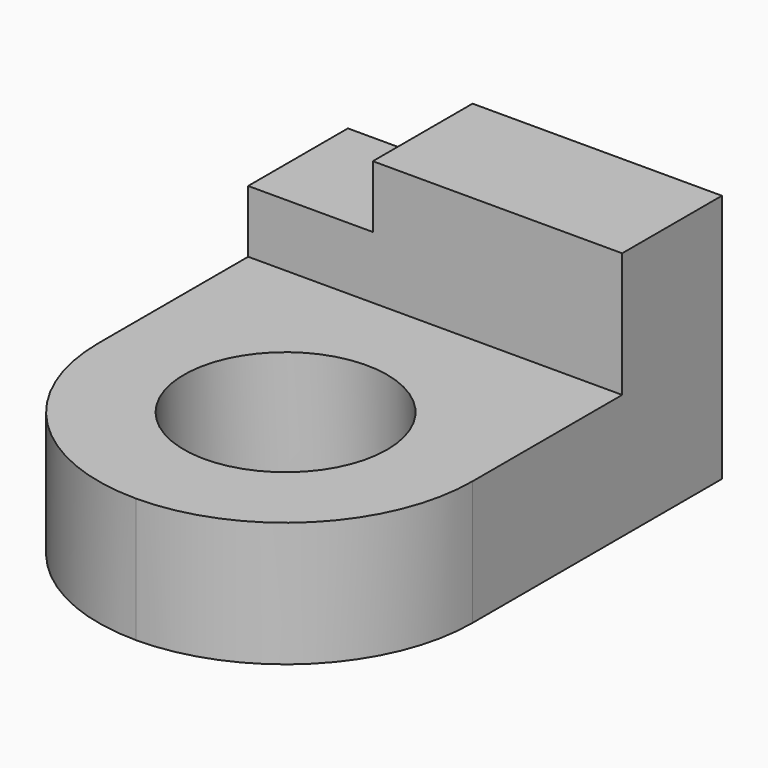
from build123d import *

# Parameters (mm, degrees)
F1_W     = 25.4
F1_H     = 12.7
F2_DEPTH = 25.4
F0_W     = 38.1
F0_H     = 50.8
F3_DEPTH = 12.7
F4_R     = 10.3422808599
F5_DEPTH = 12.701
F6_R     = 19.04999
F7_W     = 12.7
F7_H     = 6.35
F8_DEPTH = 12.7


# Not quite as in the source:
# - a fillet or chamfer is up to 0.001 mm smaller than in the source, because OpenCascade refuses the exact size


with BuildPart() as f2:
    # F1 (on face) → F2 (new body)
    with BuildSketch(Plane.XY):
        with Locations((6.35, 19.05)):
            Rectangle(F1_W, F1_H)
    extrude(amount=F2_DEPTH)

    # F0 (on Top) → F3 (join)
    with BuildSketch(Plane.XY):
        Rectangle(F0_W, F0_H)
    extrude(amount=F3_DEPTH)

    # F4 (on face) → F5 (cut, through all)
    with BuildSketch(Plane.XY.offset(12.7)):
        with Locations((0, -6.35)):
            Circle(F4_R)
    extrude(amount=-F5_DEPTH, mode=Mode.SUBTRACT)

    # F6 (radius 19.05 in the source; OpenCascade refuses exactly that, so slightly less here)
    f6_edges = [f2.edges().sort_by_distance(p)[0] for p in [
        (-19.05, -25.4, 6.35),
        (19.05, -25.4, 6.35),
    ]]
    fillet(f6_edges, radius=F6_R)

    # F7 (on face) → F8 (join)
    with BuildSketch(Plane(origin=(-6.35, 0, 0), x_dir=(0, -1, 0), z_dir=(-1, 0, 0))):
        with Locations((-19.05, 15.875)):
            Rectangle(F7_W, F7_H)
    extrude(amount=F8_DEPTH)


solid = f2.part
